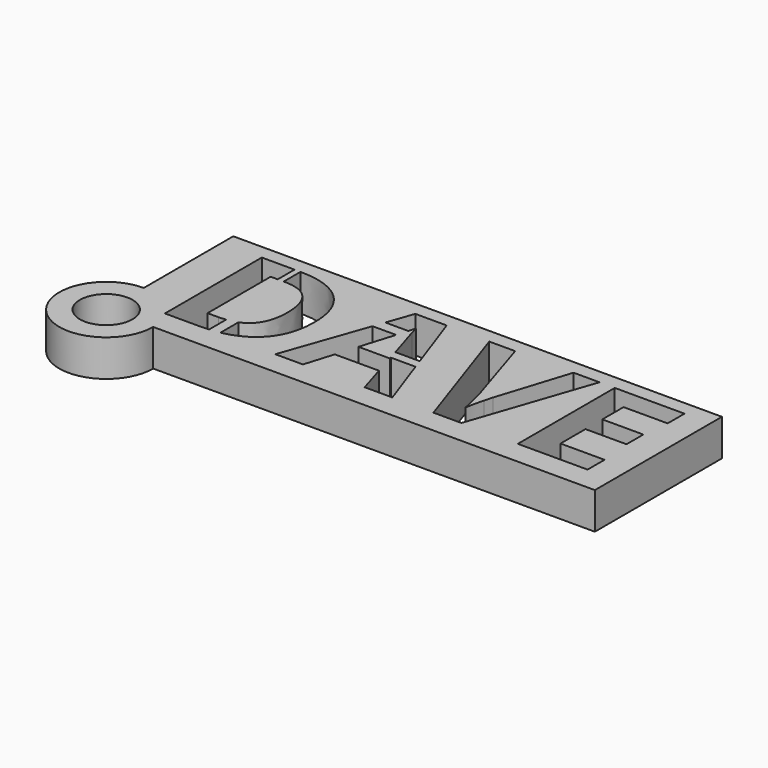
from build123d import *

# Parameters (mm, degrees)
F0_R     = 2.1552668946
F1_DEPTH = 3
F2_DEPTH = 3
F3_DEPTH = 3


# Not quite as in the source:
# - a feature names something its author has since deleted; it is built from what else it names


with BuildPart() as f1:
    # F0 (on Top) → F1 (new body)
    with BuildSketch(Plane.XY):
        with BuildLine():
            Line((8.9158927649, 2.3191112205), (-31.0841072351, 2.3191112205))
            Line((-31.0841072351, 2.3191112205), (-31.0841072351, -6.8367764676))
            ThreePointArc((-31.0841072351, -6.8367764676), (-29.2190156428, -7.3195448787), (-27.8223845073, -8.6465917722))
            Line((-27.8223845073, -8.6465917722), (-27.8223845073, 1.160879073))
            Line((-27.8223845073, 1.160879073), (-25.1418892294, 1.160879073))
            Line((-25.1418892294, 1.160879073), (-24.7104053406, 1.160879073))
            add(Edge.make_bspline(
                [(-24.7104053406, 1.160879073), (-24.680544405, 1.160879073), (-24.6508475393, 1.1606853064)],
                knots=[0, 0, 0, 0.0122966212, 0.0122966212, 0.0122966212], degree=2))
            add(Edge.make_bspline(
                [(-24.6508475393, 1.1606853064), (-22.2655016763, 1.1451213586), (-20.9387039517, -0.1205879408)],
                knots=[0.0122966212, 0.0122966212, 0.0122966212, 1, 1, 1], degree=2))
            add(Edge.make_bspline(
                [(-20.9387039517, -0.1205879408), (-19.5953879795, -1.4020549547), (-19.5953879795, -3.702402177)],
                knots=[0, 0, 0, 1, 1, 1], degree=2))
            add(Edge.make_bspline(
                [(-19.5953879795, -3.702402177), (-19.5953879795, -6.1503188436), (-20.9897022156, -7.452402177)],
                knots=[0, 0, 0, 1, 1, 1], degree=2))
            add(Edge.make_bspline(
                [(-20.9897022156, -7.452402177), (-21.9161308918, -8.3175495789), (-23.3881715685, -8.60786432)],
                knots=[0, 0, 0, 0.6644332047, 0.6644332047, 0.6644332047], degree=2))
            add(Edge.make_bspline(
                [(-23.3881715685, -8.60786432), (-23.7888512634, -8.6868860643), (-24.2299549282, -8.7233189027)],
                knots=[0.6644332047, 0.6644332047, 0.6644332047, 0.8452875098, 0.8452875098, 0.8452875098], degree=2))
            add(Edge.make_bspline(
                [(-24.2299549282, -8.7233189027), (-24.6072987041, -8.7544855103), (-25.0142247851, -8.7544855103)],
                knots=[0.8452875098, 0.8452875098, 0.8452875098, 1, 1, 1], degree=2))
            Line((-25.0142247851, -8.7544855103), (-27.7575219121, -8.7544855103))
            ThreePointArc((-27.7575219121, -8.7544855103), (-27.3716304969, -9.6835343114), (-27.2399949232, -10.6808887795))
            Line((-27.2399949232, -10.6808887795), (8.9158927649, -10.6808887795))
            Line((8.9158927649, -10.6808887795), (8.9158927649, 2.3191112205))
        make_face()
        Polygon((-10.9760084531, -3.7350449711), (-10.7037159156, -4.5066806488), (-9.2047629795, -8.7544855103), (-11.4703879795, -8.7544855103), (-12.1887039517, -6.3933743992), (-15.8041553406, -6.3933743992), (-16.5224713128, -8.7544855103), (-18.7880963128, -8.7544855103), (-16.3575375911, -1.8410302), (-16.0369298862, -0.9290970629), (-15.2876622851, 1.2021117119), (-12.7182178406, 1.2021117119), align=None, mode=Mode.SUBTRACT)
        with BuildLine():
            Line((-0.1791553406, 1.160879073), (-2.8697243415, -6.7549031323))
            Line((-2.8697243415, -6.7549031323), (-3.0723898417, -7.3511546909))
            Line((-3.0723898417, -7.3511546909), (-3.5493810351, -8.7544855103))
            Line((-3.5493810351, -8.7544855103), (-5.8410477017, -8.7544855103))
            Line((-5.8410477017, -8.7544855103), (-9.2047629795, 1.160879073))
            Line((-9.2047629795, 1.160879073), (-7.0823671462, 1.160879073))
            Line((-7.0823671462, 1.160879073), (-5.2160477017, -4.7397285658))
            add(Edge.make_bspline(
                [(-5.2160477017, -4.7397285658), (-5.0619678406, -5.2627320381), (-4.8948671462, -5.9571764825)],
                knots=[0, 0, 0, 1, 1, 1], degree=2))
            add(Edge.make_bspline(
                [(-4.8948671462, -5.9571764825), (-4.7277664517, -6.651620927), (-4.6887039517, -6.9228882881)],
                knots=[0, 0, 0, 1, 1, 1], degree=2))
            add(Edge.make_bspline(
                [(-4.6887039517, -6.9228882881), (-4.6303623692, -6.4444873114), (-4.360761049, -5.4129699306)],
                knots=[0, 0, 0, 0.7681086064, 0.7681086064, 0.7681086064], degree=2))
            add(Edge.make_bspline(
                [(-4.360761049, -5.4129699306), (-4.2793686191, -5.1015556319), (-4.1787213128, -4.7397285658)],
                knots=[0.7681086064, 0.7681086064, 0.7681086064, 1, 1, 1], degree=2))
            Line((-4.1787213128, -4.7397285658), (-2.301551174, 1.160879073))
            Line((-2.301551174, 1.160879073), (-0.1791553406, 1.160879073))
        make_face(mode=Mode.SUBTRACT)
        Polygon((6.7783099372, -7.0183743992), (6.7783099372, -8.7544855103), (1.0686745205, -8.7544855103), (1.0686745205, 1.160879073), (6.7783099372, 1.160879073), (6.7783099372, -0.5622112047), (3.1715391038, -0.5622112047), (3.1715391038, -2.7388605103), (6.5287439649, -2.7388605103), (6.5287439649, -4.4619507881), (3.1715391038, -4.4619507881), (3.1715391038, -7.0183743992), align=None, mode=Mode.SUBTRACT)
        with BuildLine():
            ThreePointArc((-27.8223845073, -8.6465917722), (-29.2190156428, -7.3195448787), (-31.0841072351, -6.8367764676))
            ThreePointArc((-31.0841072351, -6.8367764676), (-33.8023051185, -13.3990866629), (-27.2399949232, -10.6808887795))
            ThreePointArc((-27.2399949232, -10.6808887795), (-27.3716304969, -9.6835343114), (-27.7575219121, -8.7544855103))
            Line((-27.7575219121, -8.7544855103), (-27.8223845073, -8.7544855103))
            Line((-27.8223845073, -8.7544855103), (-27.8223845073, -8.6465917722))
        make_face()
        with Locations((-31.0841072351, -10.6808887795)):
            Circle(F0_R, mode=Mode.SUBTRACT)
        with BuildLine():
            Line((-24.6508475393, -0.5622112047), (-25.1418892294, -0.5622112047))
            Line((-25.1418892294, -0.5622112047), (-25.719519924, -0.5622112047))
            Line((-25.719519924, -0.5622112047), (-25.719519924, -7.0183743992))
            Line((-25.719519924, -7.0183743992), (-24.8189122851, -7.0183743992))
            add(Edge.make_bspline(
                [(-24.8189122851, -7.0183743992), (-24.5085848668, -7.0183743992), (-24.2299549282, -6.9843448907)],
                knots=[0, 0, 0, 0.1021420531, 0.1021420531, 0.1021420531], degree=2))
            add(Edge.make_bspline(
                [(-24.2299549282, -6.9843448907), (-23.7649142238, -6.9275487449), (-23.3881715685, -6.7759583364)],
                knots=[0.1021420531, 0.1021420531, 0.1021420531, 0.2726198293, 0.2726198293, 0.2726198293], degree=2))
            add(Edge.make_bspline(
                [(-23.3881715685, -6.7759583364), (-21.7807178406, -6.1291651903), (-21.7807178406, -3.7566556492)],
                knots=[0.2726198293, 0.2726198293, 0.2726198293, 1, 1, 1], degree=2))
            add(Edge.make_bspline(
                [(-21.7807178406, -3.7566556492), (-21.7807178406, -0.5622112047), (-24.6018983962, -0.5622112047)],
                knots=[0, 0, 0, 1, 1, 1], degree=2))
            Line((-24.6018983962, -0.5622112047), (-24.6508475393, -0.5622112047))
        make_face()
        with BuildLine():
            add(Edge.make_bspline(
                [(-12.692176174, -4.6312216214), (-12.7116804628, -4.5684169616), (-12.7308511011, -4.5066806488)],
                knots=[0, 0, 0, 0.0195807762, 0.0195807762, 0.0195807762], degree=2))
            add(Edge.make_bspline(
                [(-12.7308511011, -4.5066806488), (-12.8579477675, -4.0973839213), (-12.9703792713, -3.7350449711)],
                knots=[0.0195807762, 0.0195807762, 0.0195807762, 0.1493965567, 0.1493965567, 0.1493965567], degree=2))
            add(Edge.make_bspline(
                [(-12.9703792713, -3.7350449711), (-13.7070741781, -1.3608593558), (-13.8141379795, -1.0027493992)],
                knots=[0.1493965567, 0.1493965567, 0.1493965567, 1, 1, 1], degree=2))
            add(Edge.make_bspline(
                [(-13.8141379795, -1.0027493992), (-13.9400060351, -0.5817424547), (-13.9942595073, -0.3386868992)],
                knots=[0, 0, 0, 1, 1, 1], degree=2))
            add(Edge.make_bspline(
                [(-13.9942595073, -0.3386868992), (-14.0498886573, -0.5547224332), (-14.1571325889, -0.9290970629)],
                knots=[0, 0, 0, 0.2488729353, 0.2488729353, 0.2488729353], degree=2))
            add(Edge.make_bspline(
                [(-14.1571325889, -0.9290970629), (-14.2648638581, -1.3051729247), (-14.4246800702, -1.8410302)],
                knots=[0.2488729353, 0.2488729353, 0.2488729353, 0.4988767982, 0.4988767982, 0.4988767982], degree=2))
            add(Edge.make_bspline(
                [(-14.4246800702, -1.8410302), (-14.7450255679, -2.915135657), (-15.2746414517, -4.6312216214)],
                knots=[0.4988767982, 0.4988767982, 0.4988767982, 1, 1, 1], degree=2))
            Line((-15.2746414517, -4.6312216214), (-12.692176174, -4.6312216214))
        make_face()
        with BuildLine():
            Line((-16.3575375911, -1.8410302), (-14.4246800702, -1.8410302))
            add(Edge.make_bspline(
                [(-14.1571325889, -0.9290970629), (-14.2648638581, -1.3051729247), (-14.4246800702, -1.8410302)],
                knots=[0.2488729353, 0.2488729353, 0.2488729353, 0.4988767982, 0.4988767982, 0.4988767982], degree=2))
            Line((-14.1571325889, -0.9290970629), (-16.0369298862, -0.9290970629))
            Line((-16.0369298862, -0.9290970629), (-16.3575375911, -1.8410302))
        make_face()
        with BuildLine():
            add(Edge.make_bspline(
                [(-12.7308511011, -4.5066806488), (-12.8579477675, -4.0973839213), (-12.9703792713, -3.7350449711)],
                knots=[0.0195807762, 0.0195807762, 0.0195807762, 0.1493965567, 0.1493965567, 0.1493965567], degree=2))
            Line((-12.7308511011, -4.5066806488), (-10.7037159156, -4.5066806488))
            Line((-10.7037159156, -4.5066806488), (-10.9760084531, -3.7350449711))
            Line((-10.9760084531, -3.7350449711), (-12.9703792713, -3.7350449711))
        make_face()
        with BuildLine():
            Line((-24.2299549282, -6.9843448907), (-24.2299549282, -8.7233189027))
            add(Edge.make_bspline(
                [(-23.3881715685, -8.60786432), (-23.7888512634, -8.6868860643), (-24.2299549282, -8.7233189027)],
                knots=[0.6644332047, 0.6644332047, 0.6644332047, 0.8452875098, 0.8452875098, 0.8452875098], degree=2))
            Line((-23.3881715685, -8.60786432), (-23.3881715685, -6.7759583364))
            add(Edge.make_bspline(
                [(-24.2299549282, -6.9843448907), (-23.7649142238, -6.9275487449), (-23.3881715685, -6.7759583364)],
                knots=[0.1021420531, 0.1021420531, 0.1021420531, 0.2726198293, 0.2726198293, 0.2726198293], degree=2))
        make_face()
        with BuildLine():
            Line((-24.7104053406, 1.160879073), (-25.1418892294, 1.160879073))
            Line((-25.1418892294, 1.160879073), (-25.1418892294, -0.5622112047))
            Line((-25.1418892294, -0.5622112047), (-24.6508475393, -0.5622112047))
            Line((-24.6508475393, -0.5622112047), (-24.6508475393, 1.1606853064))
            add(Edge.make_bspline(
                [(-24.7104053406, 1.160879073), (-24.680544405, 1.160879073), (-24.6508475393, 1.1606853064)],
                knots=[0, 0, 0, 0.0122966212, 0.0122966212, 0.0122966212], degree=2))
        make_face()
    extrude(amount=F1_DEPTH)

    # F0 (on Top) → F2 (join)
    with BuildSketch(Plane.XY):
        with BuildLine():
            ThreePointArc((-27.8223845073, -8.6465917722), (-29.2190156428, -7.3195448787), (-31.0841072351, -6.8367764676))
            ThreePointArc((-31.0841072351, -6.8367764676), (-33.8023051185, -13.3990866629), (-27.2399949232, -10.6808887795))
            ThreePointArc((-27.2399949232, -10.6808887795), (-27.3716304969, -9.6835343114), (-27.7575219121, -8.7544855103))
            Line((-27.7575219121, -8.7544855103), (-27.8223845073, -8.7544855103))
            Line((-27.8223845073, -8.7544855103), (-27.8223845073, -8.6465917722))
        make_face()
        with Locations((-31.0841072351, -10.6808887795)):
            Circle(F0_R, mode=Mode.SUBTRACT)
    extrude(amount=F2_DEPTH)

    # F0 (on Top) → F3 (join)
    with BuildSketch(Plane.XY):
        with BuildLine():
            Line((8.9158927649, 2.3191112205), (-31.0841072351, 2.3191112205))
            Line((-31.0841072351, 2.3191112205), (-31.0841072351, -6.8367764676))
            ThreePointArc((-31.0841072351, -6.8367764676), (-29.2190156428, -7.3195448787), (-27.8223845073, -8.6465917722))
            Line((-27.8223845073, -8.6465917722), (-27.8223845073, 1.160879073))
            Line((-27.8223845073, 1.160879073), (-25.1418892294, 1.160879073))
            Line((-25.1418892294, 1.160879073), (-24.7104053406, 1.160879073))
            add(Edge.make_bspline(
                [(-24.7104053406, 1.160879073), (-24.680544405, 1.160879073), (-24.6508475393, 1.1606853064)],
                knots=[0, 0, 0, 0.0122966212, 0.0122966212, 0.0122966212], degree=2))
            add(Edge.make_bspline(
                [(-24.6508475393, 1.1606853064), (-22.2655016763, 1.1451213586), (-20.9387039517, -0.1205879408)],
                knots=[0.0122966212, 0.0122966212, 0.0122966212, 1, 1, 1], degree=2))
            add(Edge.make_bspline(
                [(-20.9387039517, -0.1205879408), (-19.5953879795, -1.4020549547), (-19.5953879795, -3.702402177)],
                knots=[0, 0, 0, 1, 1, 1], degree=2))
            add(Edge.make_bspline(
                [(-19.5953879795, -3.702402177), (-19.5953879795, -6.1503188436), (-20.9897022156, -7.452402177)],
                knots=[0, 0, 0, 1, 1, 1], degree=2))
            add(Edge.make_bspline(
                [(-20.9897022156, -7.452402177), (-21.9161308918, -8.3175495789), (-23.3881715685, -8.60786432)],
                knots=[0, 0, 0, 0.6644332047, 0.6644332047, 0.6644332047], degree=2))
            add(Edge.make_bspline(
                [(-23.3881715685, -8.60786432), (-23.7888512634, -8.6868860643), (-24.2299549282, -8.7233189027)],
                knots=[0.6644332047, 0.6644332047, 0.6644332047, 0.8452875098, 0.8452875098, 0.8452875098], degree=2))
            add(Edge.make_bspline(
                [(-24.2299549282, -8.7233189027), (-24.6072987041, -8.7544855103), (-25.0142247851, -8.7544855103)],
                knots=[0.8452875098, 0.8452875098, 0.8452875098, 1, 1, 1], degree=2))
            Line((-25.0142247851, -8.7544855103), (-27.7575219121, -8.7544855103))
            ThreePointArc((-27.7575219121, -8.7544855103), (-27.3716304969, -9.6835343114), (-27.2399949232, -10.6808887795))
            Line((-27.2399949232, -10.6808887795), (8.9158927649, -10.6808887795))
            Line((8.9158927649, -10.6808887795), (8.9158927649, 2.3191112205))
        make_face()
        Polygon((-10.9760084531, -3.7350449711), (-10.7037159156, -4.5066806488), (-9.2047629795, -8.7544855103), (-11.4703879795, -8.7544855103), (-12.1887039517, -6.3933743992), (-15.8041553406, -6.3933743992), (-16.5224713128, -8.7544855103), (-18.7880963128, -8.7544855103), (-16.3575375911, -1.8410302), (-16.0369298862, -0.9290970629), (-15.2876622851, 1.2021117119), (-12.7182178406, 1.2021117119), align=None, mode=Mode.SUBTRACT)
        with BuildLine():
            Line((-0.1791553406, 1.160879073), (-2.8697243415, -6.7549031323))
            Line((-2.8697243415, -6.7549031323), (-3.0723898417, -7.3511546909))
            Line((-3.0723898417, -7.3511546909), (-3.5493810351, -8.7544855103))
            Line((-3.5493810351, -8.7544855103), (-5.8410477017, -8.7544855103))
            Line((-5.8410477017, -8.7544855103), (-9.2047629795, 1.160879073))
            Line((-9.2047629795, 1.160879073), (-7.0823671462, 1.160879073))
            Line((-7.0823671462, 1.160879073), (-5.2160477017, -4.7397285658))
            add(Edge.make_bspline(
                [(-5.2160477017, -4.7397285658), (-5.0619678406, -5.2627320381), (-4.8948671462, -5.9571764825)],
                knots=[0, 0, 0, 1, 1, 1], degree=2))
            add(Edge.make_bspline(
                [(-4.8948671462, -5.9571764825), (-4.7277664517, -6.651620927), (-4.6887039517, -6.9228882881)],
                knots=[0, 0, 0, 1, 1, 1], degree=2))
            add(Edge.make_bspline(
                [(-4.6887039517, -6.9228882881), (-4.6303623692, -6.4444873114), (-4.360761049, -5.4129699306)],
                knots=[0, 0, 0, 0.7681086064, 0.7681086064, 0.7681086064], degree=2))
            add(Edge.make_bspline(
                [(-4.360761049, -5.4129699306), (-4.2793686191, -5.1015556319), (-4.1787213128, -4.7397285658)],
                knots=[0.7681086064, 0.7681086064, 0.7681086064, 1, 1, 1], degree=2))
            Line((-4.1787213128, -4.7397285658), (-2.301551174, 1.160879073))
            Line((-2.301551174, 1.160879073), (-0.1791553406, 1.160879073))
        make_face(mode=Mode.SUBTRACT)
        Polygon((6.7783099372, -7.0183743992), (6.7783099372, -8.7544855103), (1.0686745205, -8.7544855103), (1.0686745205, 1.160879073), (6.7783099372, 1.160879073), (6.7783099372, -0.5622112047), (3.1715391038, -0.5622112047), (3.1715391038, -2.7388605103), (6.5287439649, -2.7388605103), (6.5287439649, -4.4619507881), (3.1715391038, -4.4619507881), (3.1715391038, -7.0183743992), align=None, mode=Mode.SUBTRACT)
        with BuildLine():
            ThreePointArc((-27.8223845073, -8.6465917722), (-29.2190156428, -7.3195448787), (-31.0841072351, -6.8367764676))
            ThreePointArc((-31.0841072351, -6.8367764676), (-33.8023051185, -13.3990866629), (-27.2399949232, -10.6808887795))
            ThreePointArc((-27.2399949232, -10.6808887795), (-27.3716304969, -9.6835343114), (-27.7575219121, -8.7544855103))
            Line((-27.7575219121, -8.7544855103), (-27.8223845073, -8.7544855103))
            Line((-27.8223845073, -8.7544855103), (-27.8223845073, -8.6465917722))
        make_face()
        with Locations((-31.0841072351, -10.6808887795)):
            Circle(F0_R, mode=Mode.SUBTRACT)
    extrude(amount=F3_DEPTH)


solid = f1.part
